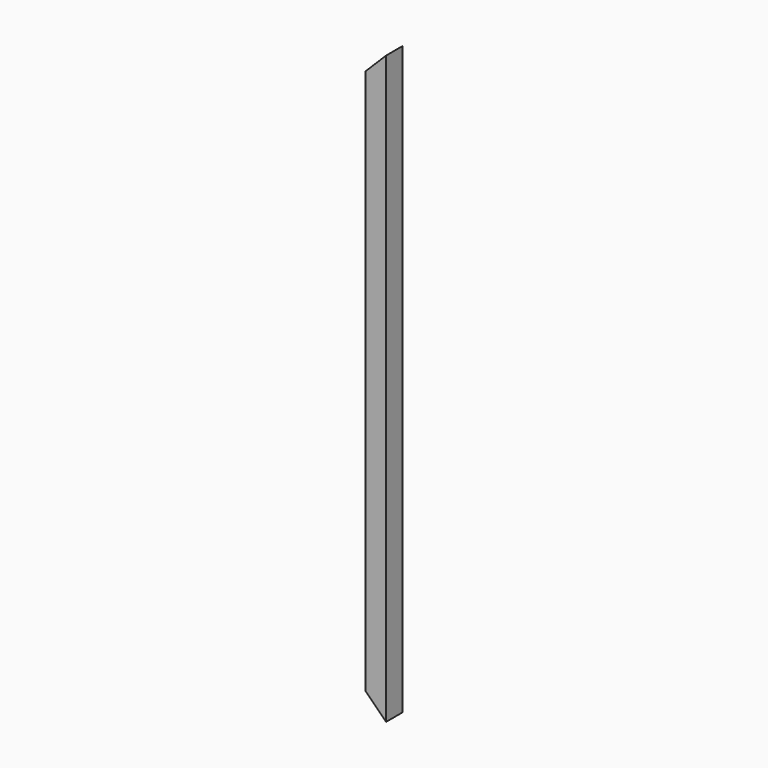
from build123d import *

# Parameters (mm, degrees)
F0_W        = 50
F0_H        = 50
F0_W_2      = 44
F0_H_2      = 44
F1_DEPTH    = 1430
F2_T1_DEPTH = 307.1682987966


# Not quite as in the source:
# - a fillet or chamfer that OpenCascade refuses, or shapes differently, is made with other operations: its cross-section is extruded or revolved along the edge and cut away or added


with BuildPart() as f1:
    # F0 (on Top) → F1 (new body)
    with BuildSketch(Plane.XY):
        with Locations((25, 25)):
            Rectangle(F0_W, F0_H)
        with Locations((25, 25)):
            Rectangle(F0_W_2, F0_H_2, mode=Mode.SUBTRACT)
    extrude(amount=F1_DEPTH)

    # F2: chamfer of 50 on 2 edges, made by hand

    # F2_s2 → F2_t1 (cut)
    with BuildSketch(Plane.XZ.offset(-178.5841493983)):
        Polygon((0, 50), (50, 0), (0, 0), align=None)
        Polygon((0, 1380), (50, 1430), (0, 1430), align=None)
    extrude(amount=F2_T1_DEPTH, mode=Mode.SUBTRACT)


solid = f1.part
